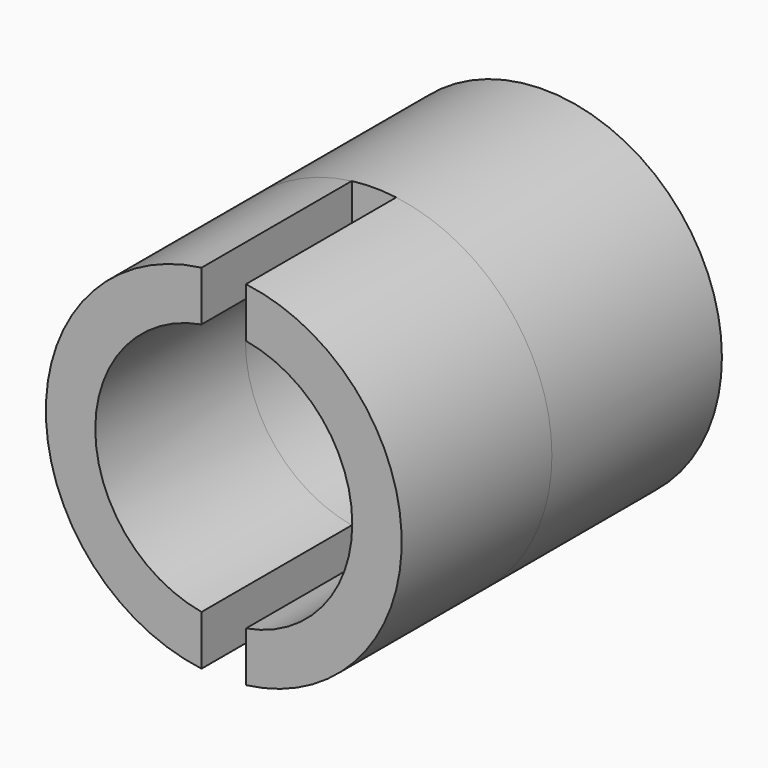
from build123d import *
from build123d import SkipClean  # not in build123d's __all__

# Parameters (mm, degrees)
F0_R     = 9.144
F0_R_2   = 6.604
F1_DEPTH = 10.922
F4_DEPTH = 9.652


with BuildPart() as f1:
    # F0 (on Front) → F1 (new body)
    with BuildSketch(Plane.XZ):
        Circle(F0_R)
        Circle(F0_R_2, mode=Mode.SUBTRACT)
    extrude(amount=F1_DEPTH)

    # F3 (on offset) → F4 (join)
    with BuildSketch(Plane.XZ.offset(20.574)):
        with BuildLine():
            Line((-1.143, 6.5043344779), (-1.143, 9.0722812456))
            ThreePointArc((-1.143, 9.0722812456), (-9.144, 0), (-1.143, -9.0722812456))
            Line((-1.143, -9.0722812456), (-1.143, -6.5043344779))
            ThreePointArc((-1.143, -6.5043344779), (-6.604, 0), (-1.143, 6.5043344779))
        make_face()
        with BuildLine():
            ThreePointArc((1.143, -9.0722812456), (9.144, 0), (1.143, 9.0722812456))
            Line((1.143, 9.0722812456), (1.143, 6.5043344779))
            ThreePointArc((1.143, 6.5043344779), (6.604, 0), (1.143, -6.5043344779))
            Line((1.143, -6.5043344779), (1.143, -9.0722812456))
        make_face()
    with SkipClean():  # cleaning this boolean's faces spoils the solid; the shape is the same uncleaned
        extrude(amount=-F4_DEPTH)


solid = f1.part
